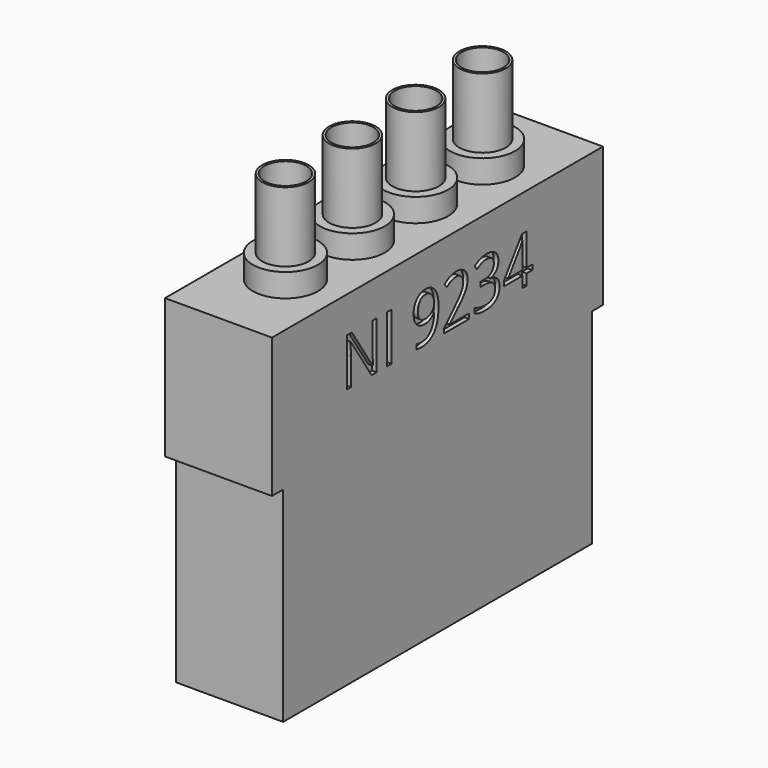
from build123d import *

# Parameters (mm, degrees)
F1_DEPTH     = 23
F2_R         = 5
F2_R_2       = 4.5
F3_DEPTH     = 20
F4_R         = 7
F5_DEPTH     = 5
F6_TEXT_SIZE = 14.4042281641
F7_DEPTH     = 1


# Not quite as in the source:
# - Text() gives the source's letters only with a copy of the font that has no kerning and outlines rounded to 1/6400 em; it was checked with that copy


with BuildPart() as f1:
    # F0 (on Right) → F1 (new body)
    with BuildSketch(Plane.YZ):
        Polygon((0, 44), (0, 0), (83, 0), (83, 44), (86, 44), (86, 74), (-3, 74), (-3, 44), align=None)
    extrude(amount=F1_DEPTH)

    # F2 (on face) → F3 (join)
    with BuildSketch(Plane.XY.offset(74)):
        with Locations((11.5, 15)):
            Circle(F2_R)
        with Locations((11.5, 15)):
            Circle(F2_R_2, mode=Mode.SUBTRACT)
        with Locations((11.5, 68)):
            Circle(F2_R)
        with Locations((11.5, 68)):
            Circle(F2_R_2, mode=Mode.SUBTRACT)
        with Locations((11.5, 50)):
            Circle(F2_R)
        with Locations((11.5, 50)):
            Circle(F2_R_2, mode=Mode.SUBTRACT)
        with Locations((11.5, 33)):
            Circle(F2_R)
        with Locations((11.5, 33)):
            Circle(F2_R_2, mode=Mode.SUBTRACT)
    extrude(amount=F3_DEPTH)

    # F4 (on face) → F5 (join)
    with BuildSketch(Plane.XY.offset(74)):
        with Locations((11.5, 68)):
            Circle(F4_R)
        with Locations((11.5, 50)):
            Circle(F4_R)
        with Locations((11.5, 33)):
            Circle(F4_R)
        with Locations((11.5, 15)):
            Circle(F4_R)
    extrude(amount=F5_DEPTH)

    # F6 (on face) → F7 (cut)
    with BuildSketch(Plane.YZ.offset(23)):
        with Locations((15.7205369323, 55.9642016888)):
            Text('NI 9234', F6_TEXT_SIZE, font='Open Sans', text_align=(TextAlign.LEFT, TextAlign.BOTTOM))
    extrude(amount=-F7_DEPTH, mode=Mode.SUBTRACT)


solid = f1.part
